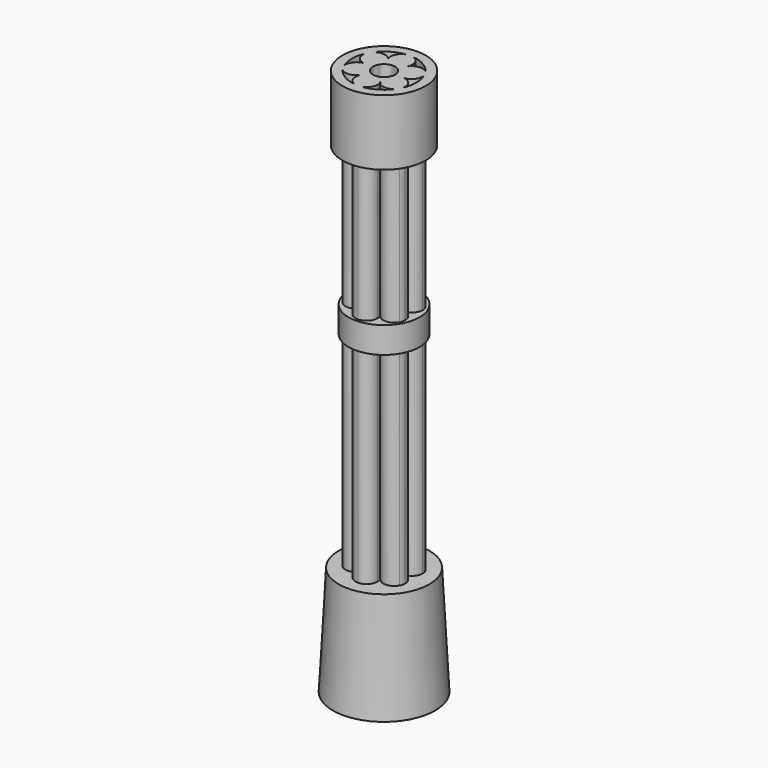
from build123d import *

# Parameters (mm, degrees)
F1_DEPTH = 25.4
F0_R     = 4.1207252188
F2_DEPTH = 1.524
F4_DEPTH = 5.08
F5_R     = 4.826
F6_DEPTH = 7.62
F8_R     = 5.2675515525
F9_DEPTH = 12.7
F9_TAPER = -3


with BuildPart() as f1:
    # F0 (on Top) → F1 (new body, symmetric)
    with BuildSketch(Plane.XY):
        with BuildLine():
            ThreePointArc((1.0998522687, -0.6349999897), (1.2267258009, -0.3287001815), (1.27, 0))
            ThreePointArc((1.27, 0), (1.2267257989, 0.328700189), (1.0998522611, 0.635000003))
            ThreePointArc((1.0998522611, 0.635000003), (0.6349999985, 1.0998522637), (0, 1.27))
            ThreePointArc((0, 1.27), (-0.6349999991, 1.0998522633), (-1.0998522618, 0.6350000018))
            ThreePointArc((-1.0998522618, 0.6350000018), (-1.27, 3.4e-09), (-1.0998522652, -0.6349999959))
            ThreePointArc((-1.0998522652, -0.6349999959), (-0.6350000021, -1.0998522616), (0, -1.27))
            ThreePointArc((0, -1.27), (0.6350000051, -1.0998522598), (1.0998522687, -0.6349999897))
        make_face()
        with BuildLine():
            ThreePointArc((-1.0998522618, 0.6350000018), (-0.6349999991, 1.0998522633), (0, 1.27))
            ThreePointArc((0, 1.27), (-0.6350000007, 1.4401477376), (-1.0998522636, 1.9050000014))
            ThreePointArc((-1.0998522636, 1.9050000014), (-0.9729787264, 1.5987001881), (-0.9297045256, 1.27))
            ThreePointArc((-0.9297045256, 1.27), (-0.972978726, 0.9412998137), (-1.0998522618, 0.6350000018))
        make_face()
        with BuildLine():
            ThreePointArc((0, 1.27), (0.6349999985, 1.0998522637), (1.0998522611, 0.635000003))
            ThreePointArc((1.0998522611, 0.635000003), (0.9297045256, 1.2699999943), (1.0998522553, 1.904999987))
            ThreePointArc((1.0998522553, 1.904999987), (0.6349999935, 1.4401477334), (0, 1.27))
        make_face()
        with BuildLine():
            ThreePointArc((1.0998522611, 0.635000003), (1.2267257989, 0.328700189), (1.27, 0))
            ThreePointArc((1.27, 0), (1.2267258009, -0.3287001815), (1.0998522687, -0.6349999897))
            ThreePointArc((1.0998522687, -0.6349999897), (1.5647045337, -0.1701477325), (2.1997045323, 0))
            ThreePointArc((2.1997045323, 0), (1.564704527, 0.1701477364), (1.0998522611, 0.635000003))
        make_face()
        with BuildLine():
            ThreePointArc((1.0998522687, -1.9050000103), (0.9297045256, -1.27), (1.0998522687, -0.6349999897))
            ThreePointArc((1.0998522687, -0.6349999897), (0.6350000051, -1.0998522598), (0, -1.27))
            ThreePointArc((0, -1.27), (0.6350000051, -1.4401477402), (1.0998522687, -1.9050000103))
        make_face()
        with BuildLine():
            ThreePointArc((-1.0998522652, -1.9050000041), (-0.635000002, -1.4401477384), (0, -1.27))
            ThreePointArc((0, -1.27), (-0.6350000021, -1.0998522616), (-1.0998522652, -0.6349999959))
            ThreePointArc((-1.0998522652, -0.6349999959), (-0.9729787268, -0.9412998104), (-0.9297045256, -1.27))
            ThreePointArc((-0.9297045256, -1.27), (-0.9729787268, -1.5987001896), (-1.0998522652, -1.9050000041))
        make_face()
        with BuildLine():
            ThreePointArc((-1.0998522652, -0.6349999959), (-1.27, 3.4e-09), (-1.0998522618, 0.6350000018))
            ThreePointArc((-1.0998522618, 0.6350000018), (-1.5647045247, 0.1701477377), (-2.1997045256, 0))
            ThreePointArc((-2.1997045256, 0), (-1.5647045277, -0.170147736), (-1.0998522652, -0.6349999959))
        make_face()
        with BuildLine():
            ThreePointArc((-1.0998522636, 1.9050000014), (-0.6350000007, 1.4401477376), (0, 1.27))
            ThreePointArc((0, 1.27), (0.6349999935, 1.4401477334), (1.0998522553, 1.904999987))
            ThreePointArc((1.0998522553, 1.904999987), (1.2267257974, 2.2112998055), (1.27, 2.54))
            ThreePointArc((1.27, 2.54), (0.8980256121, 3.4380256121), (0, 3.81))
            ThreePointArc((0, 3.81), (-1.0998522624, 3.1750000007), (-1.0998522636, 1.9050000014))
        make_face()
        with BuildLine():
            ThreePointArc((-2.1997045256, 0), (-1.5647045247, 0.1701477377), (-1.0998522618, 0.6350000018))
            ThreePointArc((-1.0998522618, 0.6350000018), (-0.972978726, 0.9412998137), (-0.9297045256, 1.27))
            ThreePointArc((-0.9297045256, 1.27), (-0.9729787264, 1.5987001881), (-1.0998522636, 1.9050000014))
            ThreePointArc((-1.0998522636, 1.9050000014), (-2.1997045238, 2.54), (-3.2995567858, 1.9050000045))
            ThreePointArc((-3.2995567858, 1.9050000045), (-3.2995567897, 0.6350000022), (-2.1997045256, 0))
        make_face()
        with BuildLine():
            ThreePointArc((-0.9297045256, -1.27), (-0.9729787268, -0.9412998104), (-1.0998522652, -0.6349999959))
            ThreePointArc((-1.0998522652, -0.6349999959), (-1.5647045277, -0.170147736), (-2.1997045256, 0))
            ThreePointArc((-2.1997045256, 0), (-3.2995568097, -0.6350000369), (-3.2995567458, -1.9050000739))
            ThreePointArc((-3.2995567458, -1.9050000739), (-2.1997044853, -2.54), (-1.0998522652, -1.9050000041))
            ThreePointArc((-1.0998522652, -1.9050000041), (-0.9729787268, -1.5987001896), (-0.9297045256, -1.27))
        make_face()
        with BuildLine():
            ThreePointArc((1.0998522687, -1.9050000103), (0.6350000051, -1.4401477402), (0, -1.27))
            ThreePointArc((0, -1.27), (-0.635000002, -1.4401477384), (-1.0998522652, -1.9050000041))
            ThreePointArc((-1.0998522652, -1.9050000041), (-1.0998522616, -3.175000002), (0, -3.81))
            ThreePointArc((0, -3.81), (0.8980256121, -3.4380256121), (1.27, -2.54))
            ThreePointArc((1.27, -2.54), (1.2267258009, -2.2112998185), (1.0998522687, -1.9050000103))
        make_face()
        with BuildLine():
            ThreePointArc((2.1997045323, 0), (1.5647045337, -0.1701477325), (1.0998522687, -0.6349999897))
            ThreePointArc((1.0998522687, -0.6349999897), (0.9297045256, -1.27), (1.0998522687, -1.9050000103))
            ThreePointArc((1.0998522687, -1.9050000103), (2.1997045101, -2.54), (3.299556767, -1.9050000371))
            ThreePointArc((3.299556767, -1.9050000371), (3.4264303195, -1.598700208), (3.4697045256, -1.27))
            ThreePointArc((3.4697045256, -1.27), (3.0977301401, -0.3719743903), (2.1997045323, 0))
        make_face()
        with BuildLine():
            ThreePointArc((1.0998522553, 1.904999987), (0.9297045256, 1.2699999943), (1.0998522611, 0.635000003))
            ThreePointArc((1.0998522611, 0.635000003), (1.564704527, 0.1701477364), (2.1997045323, 0))
            ThreePointArc((2.1997045323, 0), (3.0977301401, 0.3719743903), (3.4697045256, 1.27))
            ThreePointArc((3.4697045256, 1.27), (3.4264303195, 1.598700208), (3.299556767, 1.9050000371))
            ThreePointArc((3.299556767, 1.9050000371), (2.1997044967, 2.54), (1.0998522553, 1.904999987))
        make_face()
    extrude(amount=F1_DEPTH, both=True)

    # F0 (on Top) → F2 (join, symmetric)
    with BuildSketch(Plane.XY):
        Circle(F0_R)
        with BuildLine():
            ThreePointArc((0, 3.81), (1.9049999814, 3.2995567991), (3.299556767, 1.9050000371))
            ThreePointArc((3.299556767, 1.9050000371), (3.6801773926, 0.9861005825), (3.81, 0))
            ThreePointArc((3.81, 0), (3.6801773926, -0.9861005825), (3.299556767, -1.9050000371))
            ThreePointArc((3.299556767, -1.9050000371), (1.9049999814, -3.2995567991), (0, -3.81))
            ThreePointArc((0, -3.81), (-1.9049999631, -3.2995568097), (-3.2995567458, -1.9050000739))
            ThreePointArc((-3.2995567458, -1.9050000739), (-3.81, -4.01e-08), (-3.2995567858, 1.9050000045))
            ThreePointArc((-3.2995567858, 1.9050000045), (-1.9049999978, 3.2995567897), (0, 3.81))
        make_face(mode=Mode.SUBTRACT)
        with BuildLine():
            ThreePointArc((-3.2995567858, 1.9050000045), (-2.1997045238, 2.54), (-1.0998522636, 1.9050000014))
            ThreePointArc((-1.0998522636, 1.9050000014), (-1.0998522624, 3.1750000007), (0, 3.81))
            ThreePointArc((0, 3.81), (-1.9049999978, 3.2995567897), (-3.2995567858, 1.9050000045))
        make_face()
        with BuildLine():
            ThreePointArc((1.27, 2.54), (1.2267257974, 2.2112998055), (1.0998522553, 1.904999987))
            ThreePointArc((1.0998522553, 1.904999987), (2.1997044967, 2.54), (3.299556767, 1.9050000371))
            ThreePointArc((3.299556767, 1.9050000371), (1.9049999814, 3.2995567991), (0, 3.81))
            ThreePointArc((0, 3.81), (0.8980256121, 3.4380256121), (1.27, 2.54))
        make_face()
        with BuildLine():
            ThreePointArc((3.4697045256, 1.27), (3.0977301401, 0.3719743903), (2.1997045323, 0))
            ThreePointArc((2.1997045323, 0), (3.0977301401, -0.3719743903), (3.4697045256, -1.27))
            ThreePointArc((3.4697045256, -1.27), (3.4264303195, -1.598700208), (3.299556767, -1.9050000371))
            ThreePointArc((3.299556767, -1.9050000371), (3.6801773926, -0.9861005825), (3.81, 0))
            ThreePointArc((3.81, 0), (3.6801773926, 0.9861005825), (3.299556767, 1.9050000371))
            ThreePointArc((3.299556767, 1.9050000371), (3.4264303195, 1.598700208), (3.4697045256, 1.27))
        make_face()
        with BuildLine():
            ThreePointArc((3.299556767, -1.9050000371), (2.1997045101, -2.54), (1.0998522687, -1.9050000103))
            ThreePointArc((1.0998522687, -1.9050000103), (1.2267258009, -2.2112998185), (1.27, -2.54))
            ThreePointArc((1.27, -2.54), (0.8980256121, -3.4380256121), (0, -3.81))
            ThreePointArc((0, -3.81), (1.9049999814, -3.2995567991), (3.299556767, -1.9050000371))
        make_face()
        with BuildLine():
            ThreePointArc((0, -3.81), (-1.0998522616, -3.175000002), (-1.0998522652, -1.9050000041))
            ThreePointArc((-1.0998522652, -1.9050000041), (-2.1997044853, -2.54), (-3.2995567458, -1.9050000739))
            ThreePointArc((-3.2995567458, -1.9050000739), (-1.9049999631, -3.2995568097), (0, -3.81))
        make_face()
        with BuildLine():
            ThreePointArc((-3.2995567458, -1.9050000739), (-3.2995568097, -0.6350000369), (-2.1997045256, 0))
            ThreePointArc((-2.1997045256, 0), (-3.2995567897, 0.6350000022), (-3.2995567858, 1.9050000045))
            ThreePointArc((-3.2995567858, 1.9050000045), (-3.81, -4.01e-08), (-3.2995567458, -1.9050000739))
        make_face()
    extrude(amount=F2_DEPTH, both=True)

    # F3 (on face) → F4 (cut)
    with BuildSketch(Plane.XY.offset(25.4)):
        with BuildLine():
            ThreePointArc((1.1617240994, -0.5382236443), (1.2503393833, -0.2755703193), (1.2803466618, 0))
            ThreePointArc((1.2803466618, 0), (1.2503393833, 0.2755703193), (1.1617240994, 0.5382236443))
            ThreePointArc((1.1617240994, 0.5382236443), (1.0998522628, 0.635), (1.0469773986, 0.7369707601))
            ThreePointArc((1.0469773986, 0.7369707601), (0.6401733309, 1.1088127348), (0.1147467008, 1.2751944044))
            ThreePointArc((0.1147467008, 1.2751944044), (0, 1.27), (-0.1147467008, 1.2751944044))
            ThreePointArc((-0.1147467008, 1.2751944044), (-0.6401733309, 1.1088127348), (-1.0469773986, 0.7369707601))
            ThreePointArc((-1.0469773986, 0.7369707601), (-1.0998522628, 0.635), (-1.1617240994, 0.5382236443))
            ThreePointArc((-1.1617240994, 0.5382236443), (-1.2803466618, 0), (-1.1617240994, -0.5382236443))
            ThreePointArc((-1.1617240994, -0.5382236443), (-1.0998522628, -0.635), (-1.0469773986, -0.7369707601))
            ThreePointArc((-1.0469773986, -0.7369707601), (-0.6401733309, -1.1088127348), (-0.1147467008, -1.2751944044))
            ThreePointArc((-0.1147467008, -1.2751944044), (0, -1.27), (0.1147467008, -1.2751944044))
            ThreePointArc((0.1147467008, -1.2751944044), (0.6401733309, -1.1088127348), (1.0469773986, -0.7369707601))
            ThreePointArc((1.0469773986, -0.7369707601), (1.0998522628, -0.635), (1.1617240994, -0.5382236443))
        make_face()
    extrude(amount=-F4_DEPTH, mode=Mode.SUBTRACT)

    # F5 (on face) → F6 (join)
    with BuildSketch(Plane.XY.offset(25.4)):
        Circle(F5_R)
        with BuildLine():
            ThreePointArc((0.4317572455, 3.7343557598), (2.8066798027, 2.5008749959), (3.75923227, 0))
            ThreePointArc((3.75923227, 0), (-2.5008749959, -2.8066798027), (-0.4317572455, 3.7343557598))
            ThreePointArc((-0.4317572455, 3.7343557598), (0, 3.81), (0.4317572455, 3.7343557598))
        make_face(mode=Mode.SUBTRACT)
    extrude(amount=-F6_DEPTH)

    # F8 (on offset) → F9 (join)
    with BuildSketch(Plane(origin=(0, 0, -25.4), x_dir=(1, 0, 0), z_dir=(0, 0, -1))):
        Circle(F8_R)
    extrude(amount=F9_DEPTH, taper=F9_TAPER)


solid = f1.part
